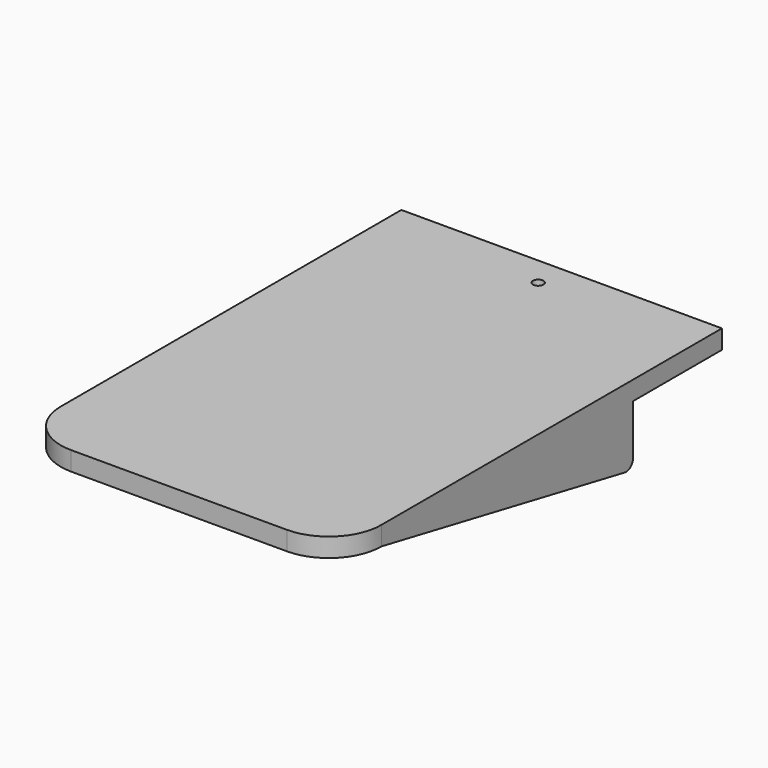
from build123d import *

# Parameters (mm, degrees)
F0_W      = 110
F0_H      = 126
F1_DEPTH  = 6.5
F2_W      = 110
F2_H      = 6.5
F3_DEPTH  = 38.1
F4_R      = 1.8
F5_DEPTH  = 14.3
F6_R      = 18
F7_R      = 18
F8_W      = 6.5
F8_H      = 146.1
F9_DEPTH  = 20.8
F10_W     = 38.1
F10_H     = 20.8
F11_DEPTH = 133.7
F13_R     = 3


# Not quite as in the source:
# - a feature of the source that left no trace in its solid (it failed there, or was rolled back) is left out


with BuildPart() as f1:
    # F0 (on Top) → F1 (new body)
    with BuildSketch(Plane.XY):
        with Locations((55, -63)):
            Rectangle(F0_W, F0_H)
    extrude(amount=F1_DEPTH)

    # F2 (on face) → F3 (join)
    with BuildSketch(Plane(origin=(0, 0, 0), x_dir=(-1, 0, 0), z_dir=(0, 1, 0))):
        with Locations((-55, 3.25)):
            Rectangle(F2_W, F2_H)
    extrude(amount=F3_DEPTH)

    # F4 (on face) → F5 (cut)
    with BuildSketch(Plane.XY.offset(6.5)):
        with Locations((55, 28.0327554792)):
            Circle(F4_R)
    extrude(amount=-F5_DEPTH, mode=Mode.SUBTRACT)

    # F6
    f6_edges = [f1.edges().sort_by_distance(p)[0] for p in [
        (110, -126, 3.25),
    ]]
    fillet(f6_edges, radius=F6_R)

    # F7
    f7_edges = [f1.edges().sort_by_distance(p)[0] for p in [
        (0, -126, 3.25),
    ]]
    fillet(f7_edges, radius=F7_R)

    # F8 (on face) → F9 (join)
    with BuildSketch(Plane(origin=(0, 0, 0), x_dir=(1, 0, 0), z_dir=(0, 0, -1))):
        with Locations((3.25, 34.95)):
            Rectangle(F8_W, F8_H)
        with Locations((106.75, 34.95)):
            Rectangle(F8_W, F8_H)
    extrude(amount=F9_DEPTH)

    # F10 (on face) → F11 (cut)
    with BuildSketch(Plane.YZ.offset(110)):
        with Locations((19.05, -10.4)):
            Rectangle(F10_W, F10_H)
        Polygon((0, -20.8), (-108, 0), (-108, -20.8), align=None)
    extrude(amount=-F11_DEPTH, mode=Mode.SUBTRACT)

    # F13
    f13_edges = [f1.edges().sort_by_distance(p)[0] for p in [
        (106.75, 0, -20.8),
        (3.25, 0, -20.8),
    ]]
    fillet(f13_edges, radius=F13_R)


solid = f1.part
